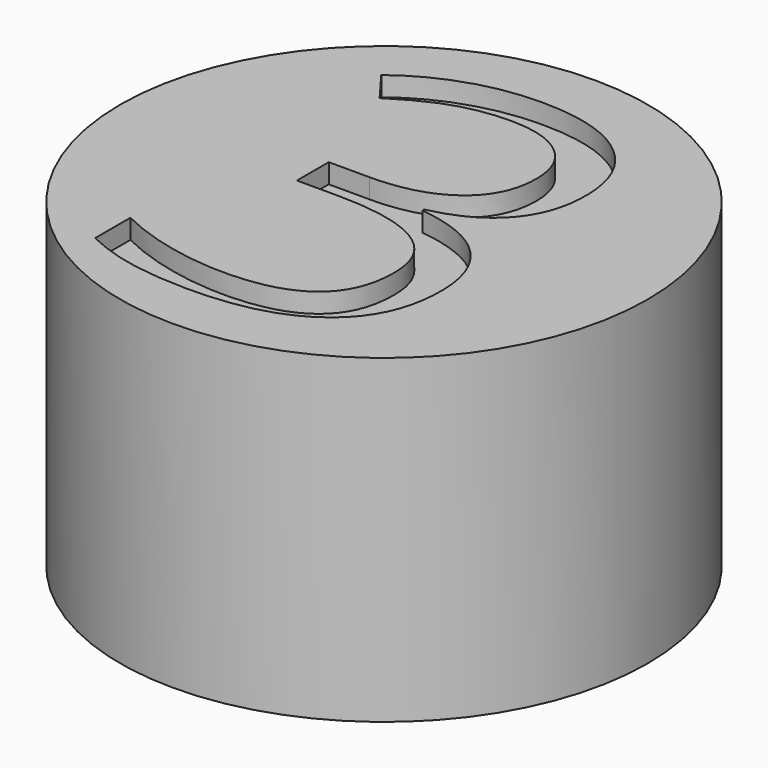
from build123d import *

# Parameters (mm, degrees)
F0_R         = 13.5
F1_DEPTH     = 16.4
F2_TEXT_SIZE = 29.2432817512
F3_DEPTH     = 1


# Not quite as in the source:
# - Text() gives the source's letters only with a copy of the font that has no kerning and outlines rounded to 1/6400 em; it was checked with that copy


with BuildPart() as f1:
    # F0 (on Top) → F1 (new body)
    with BuildSketch(Plane.XY):
        Circle(F0_R)
    extrude(amount=F1_DEPTH)

    # F2 (on face) → F3 (cut)
    with BuildSketch(Plane.XY.offset(16.4)):
        with Locations((-8.407166164, -10.4925137097)):
            Text('3', F2_TEXT_SIZE, font='Open Sans', text_align=(TextAlign.LEFT, TextAlign.BOTTOM))
    extrude(amount=-F3_DEPTH, mode=Mode.SUBTRACT)


solid = f1.part
